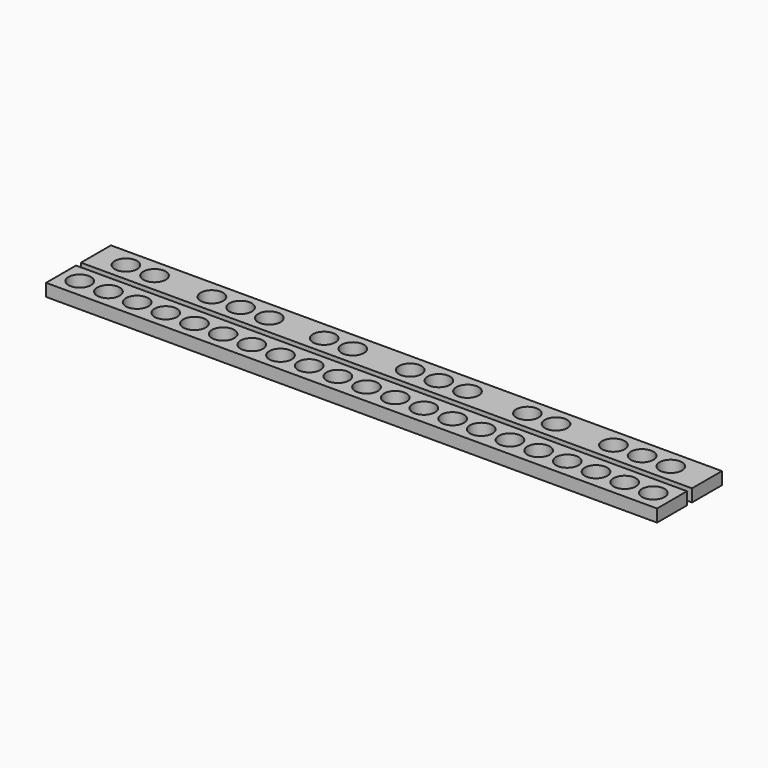
from build123d import *

# Parameters (mm, degrees)
F0_W     = 152.4
F0_H     = 50.8
F1_DEPTH = 2489.2
F2_R     = 45.72
F3_DEPTH = 63.5
F4_DEPTH = 63.5


# Not quite as in the source:
# - a feature names something its author has since deleted; it is built from what else it names


with BuildPart() as f1:
    # F0 (on Right) → F1 (new body)
    with BuildSketch(Plane.YZ):
        with Locations((0, -25.4)):
            Rectangle(F0_W, F0_H)
    extrude(amount=F1_DEPTH)

    # F2 (on Top) → F3 (cut)
    with BuildSketch(Plane.XY):
        with Locations((76.2, 0)):
            Circle(F2_R)
        with Locations((193.04, 0)):
            Circle(F2_R)
        with Locations((309.88, 0)):
            Circle(F2_R)
        with Locations((426.72, 0)):
            Circle(F2_R)
        with Locations((543.56, 0)):
            Circle(F2_R)
        with Locations((660.4, 0)):
            Circle(F2_R)
        with Locations((777.24, 0)):
            Circle(F2_R)
        with Locations((894.08, 0)):
            Circle(F2_R)
        with Locations((1010.92, 0)):
            Circle(F2_R)
        with Locations((1127.76, 0)):
            Circle(F2_R)
        with Locations((1244.6, 0)):
            Circle(F2_R)
        with Locations((1361.44, 0)):
            Circle(F2_R)
        with Locations((1595.12, 0)):
            Circle(F2_R)
        with Locations((1711.96, 0)):
            Circle(F2_R)
        with Locations((1828.8, 0)):
            Circle(F2_R)
        with Locations((1945.64, 0)):
            Circle(F2_R)
        with Locations((2062.48, 0)):
            Circle(F2_R)
        with Locations((1478.28, 0)):
            Circle(F2_R)
        with Locations((2179.32, 0)):
            Circle(F2_R)
        with Locations((2296.16, 0)):
            Circle(F2_R)
        with Locations((2413, 0)):
            Circle(F2_R)
    extrude(amount=-F3_DEPTH, mode=Mode.SUBTRACT)


with BuildPart() as f1b:
    # F0 (on Right) → F1, piece 2 (new body)
    with BuildSketch(Plane.YZ):
        with Locations((177.8, -25.4)):
            Rectangle(F0_W, F0_H)
    extrude(amount=F1_DEPTH)

    # F2 (on Top) → F4 (cut)
    with BuildSketch(Plane.XY):
        with Locations((121.92, 177.8)):
            Circle(F2_R)
        with Locations((238.76, 177.8)):
            Circle(F2_R)
        with Locations((472.44, 177.8)):
            Circle(F2_R)
        with Locations((589.28, 177.8)):
            Circle(F2_R)
        with Locations((706.12, 177.8)):
            Circle(F2_R)
        with Locations((929.64, 177.8)):
            Circle(F2_R)
        with Locations((1046.48, 177.8)):
            Circle(F2_R)
        with Locations((1280.16, 177.8)):
            Circle(F2_R)
        with Locations((1397, 177.8)):
            Circle(F2_R)
        with Locations((1513.84, 177.8)):
            Circle(F2_R)
        with Locations((1757.68, 177.8)):
            Circle(F2_R)
        with Locations((1874.52, 177.8)):
            Circle(F2_R)
        with Locations((2341.88, 177.8)):
            Circle(F2_R)
        with Locations((2225.04, 177.8)):
            Circle(F2_R)
        with Locations((2108.2, 177.8)):
            Circle(F2_R)
    extrude(amount=-F4_DEPTH, mode=Mode.SUBTRACT)


solid = Compound([f1.part, f1b.part])
